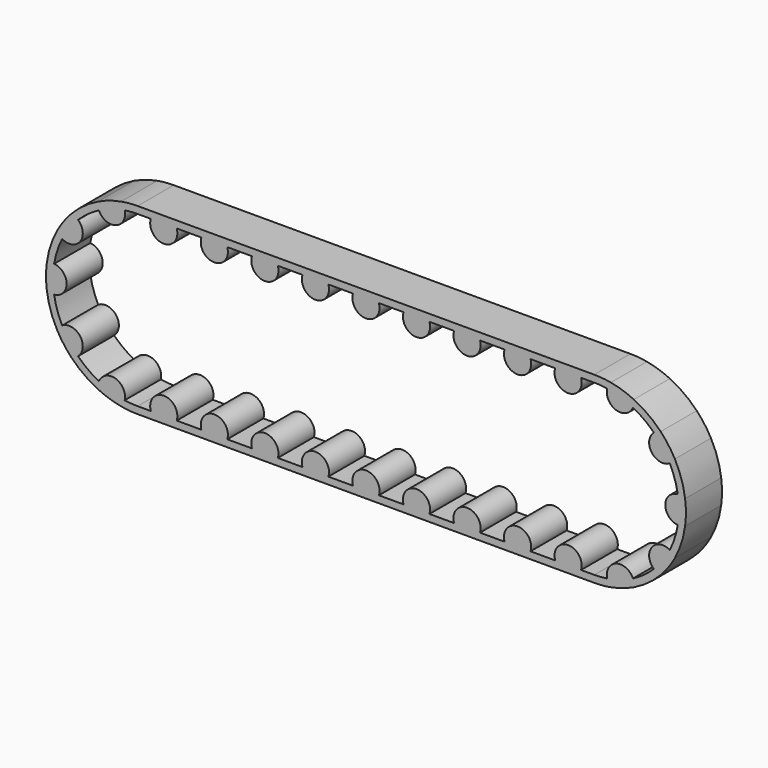
from build123d import *

# Parameters (mm, degrees)
F3_DEPTH     = 25.4
F4_TEXT_SIZE = 22.0144093166
F5_DEPTH     = 2.54


# Not quite as in the source:
# - Text() gives the source's letters only with a copy of the font that has no kerning and outlines rounded to 1/6400 em; it was checked with that copy


with BuildPart() as f3:
    # F2 (on Front) → F3 (new body)
    with BuildSketch(Plane.XZ):
        with BuildLine():
            Line((7.4325236662, -47.625), (0, -47.625))
            ThreePointArc((0, -47.625), (-3.6490858874, -47.4849954953), (-7.2767171413, -47.0658051312))
            ThreePointArc((-7.2767171413, -47.0658051312), (-8.0516506043, -49.0450507496), (-9.3413778335, -50.7345887825))
            ThreePointArc((-9.3413778335, -50.7345887825), (-4.6901126532, -51.3737547981), (0, -51.5874))
            Line((0, -51.5874), (10.3706895119, -51.5874))
            ThreePointArc((10.3706895119, -51.5874), (8.5733856685, -49.8495796433), (7.4325236662, -47.625))
        make_face()
        with BuildLine():
            ThreePointArc((-9.3413778335, -50.7345887825), (-8.0516506043, -49.0450507496), (-7.2767171413, -47.0658051312))
            ThreePointArc((-7.2767171413, -47.0658051312), (-14.7169343571, -45.2940665886), (-21.7775983128, -42.3541832258))
            ThreePointArc((-21.7775983128, -42.3541832258), (-22.3140353569, -44.4109210282), (-22.2637096494, -46.5358686543))
            ThreePointArc((-22.2637096494, -46.5358686543), (-15.9413832956, -49.0625329287), (-9.3413778335, -50.7345887825))
        make_face()
        with BuildLine():
            Line((22.001345048, -47.625), (7.4325236662, -47.625))
            ThreePointArc((7.4325236662, -47.625), (8.5733856685, -49.8495796433), (10.3706895119, -51.5874))
            Line((10.3706895119, -51.5874), (19.0631792023, -51.5874))
            ThreePointArc((19.0631792023, -51.5874), (20.8604830458, -49.8495796433), (22.001345048, -47.625))
        make_face()
        with BuildLine():
            ThreePointArc((-22.2637096494, -46.5358686543), (-22.3140353569, -44.4109210282), (-21.7775983128, -42.3541832258))
            ThreePointArc((-21.7775983128, -42.3541832258), (-27.9932726404, -38.5294343571), (-33.5515739739, -33.7998891843))
            ThreePointArc((-33.5515739739, -33.7998891843), (-35.3418797002, -34.9456380646), (-37.3783764856, -35.5544204011))
            ThreePointArc((-37.3783764856, -35.5544204011), (-30.3223129241, -41.7350832956), (-22.2637096494, -46.5358686543))
        make_face()
        with BuildLine():
            Line((35.8862447978, -47.625), (22.001345048, -47.625))
            ThreePointArc((22.001345048, -47.625), (20.8604830458, -49.8495796433), (19.0631792023, -51.5874))
            Line((19.0631792023, -51.5874), (38.8244106435, -51.5874))
            ThreePointArc((38.8244106435, -51.5874), (37.0271068, -49.8495796433), (35.8862447978, -47.625))
        make_face()
        with BuildLine():
            ThreePointArc((-37.3783764856, -35.5544204011), (-35.3418797002, -34.9456380646), (-33.5515739739, -33.7998891843))
            ThreePointArc((-33.5515739739, -33.7998891843), (-38.5294343571, -27.9932726404), (-42.5136114048, -21.4647028939))
            ThreePointArc((-42.5136114048, -21.4647028939), (-44.156518238, -22.8133289458), (-45.3648167618, -24.5620283961))
            ThreePointArc((-45.3648167618, -24.5620283961), (-41.7350832956, -30.3223129241), (-37.3783764856, -35.5544204011))
        make_face()
        with BuildLine():
            Line((50.4550661796, -47.625), (35.8862447978, -47.625))
            ThreePointArc((35.8862447978, -47.625), (37.0271068, -49.8495796433), (38.8244106435, -51.5874))
            Line((38.8244106435, -51.5874), (47.5169003339, -51.5874))
            ThreePointArc((47.5169003339, -51.5874), (49.3142041773, -49.8495796433), (50.4550661796, -47.625))
        make_face()
        with BuildLine():
            ThreePointArc((-45.3648167618, -24.5620283961), (-44.156518238, -22.8133289458), (-42.5136114048, -21.4647028939))
            ThreePointArc((-42.5136114048, -21.4647028939), (-45.2940665886, -14.7169343571), (-47.0108699246, -7.623564385))
            ThreePointArc((-47.0108699246, -7.623564385), (-49.132711977, -7.4981793975), (-51.1381057646, -6.7936718767))
            ThreePointArc((-51.1381057646, -6.7936718767), (-49.0625329287, -15.9413832956), (-45.3648167618, -24.5620283961))
        make_face()
        with BuildLine():
            Line((64.3399659294, -47.625), (50.4550661796, -47.625))
            ThreePointArc((50.4550661796, -47.625), (49.3142041773, -49.8495796433), (47.5169003339, -51.5874))
            Line((47.5169003339, -51.5874), (67.278131775, -51.5874))
            ThreePointArc((67.278131775, -51.5874), (65.4808279316, -49.8495796433), (64.3399659294, -47.625))
        make_face()
        with BuildLine():
            ThreePointArc((-51.1381057646, -6.7936718767), (-49.132711977, -7.4981793975), (-47.0108699246, -7.623564385))
            ThreePointArc((-47.0108699246, -7.623564385), (-47.625, 0), (-47.0108699246, 7.623564385))
            ThreePointArc((-47.0108699246, 7.623564385), (-49.132711977, 7.4981793975), (-51.1381057646, 6.7936718767))
            ThreePointArc((-51.1381057646, 6.7936718767), (-51.5874, 0), (-51.1381057646, -6.7936718767))
        make_face()
        with BuildLine():
            Line((78.9087873111, -47.625), (64.3399659294, -47.625))
            ThreePointArc((64.3399659294, -47.625), (65.4808279316, -49.8495796433), (67.278131775, -51.5874))
            Line((67.278131775, -51.5874), (75.9706214655, -51.5874))
            ThreePointArc((75.9706214655, -51.5874), (77.7679253089, -49.8495796433), (78.9087873111, -47.625))
        make_face()
        with BuildLine():
            ThreePointArc((-51.1381057646, 6.7936718767), (-49.132711977, 7.4981793975), (-47.0108699246, 7.623564385))
            ThreePointArc((-47.0108699246, 7.623564385), (-45.2940665886, 14.7169343571), (-42.5136114048, 21.4647028939))
            ThreePointArc((-42.5136114048, 21.4647028939), (-44.156518238, 22.8133289458), (-45.3648167618, 24.5620283961))
            ThreePointArc((-45.3648167618, 24.5620283961), (-49.0625329287, 15.9413832956), (-51.1381057646, 6.7936718767))
        make_face()
        with BuildLine():
            Line((92.7936870609, -47.625), (78.9087873111, -47.625))
            ThreePointArc((78.9087873111, -47.625), (77.7679253089, -49.8495796433), (75.9706214655, -51.5874))
            Line((75.9706214655, -51.5874), (95.7318529066, -51.5874))
            ThreePointArc((95.7318529066, -51.5874), (93.9345490632, -49.8495796433), (92.7936870609, -47.625))
        make_face()
        with BuildLine():
            ThreePointArc((-45.3648167618, 24.5620283961), (-44.156518238, 22.8133289458), (-42.5136114048, 21.4647028939))
            ThreePointArc((-42.5136114048, 21.4647028939), (-38.5294343571, 27.9932726404), (-33.5515739739, 33.7998891843))
            ThreePointArc((-33.5515739739, 33.7998891843), (-35.3418797002, 34.9456380646), (-37.3783764856, 35.5544204011))
            ThreePointArc((-37.3783764856, 35.5544204011), (-41.7350832956, 30.3223129241), (-45.3648167618, 24.5620283961))
        make_face()
        with BuildLine():
            Line((107.3625084427, -47.625), (92.7936870609, -47.625))
            ThreePointArc((92.7936870609, -47.625), (93.9345490632, -49.8495796433), (95.7318529066, -51.5874))
            Line((95.7318529066, -51.5874), (104.424342597, -51.5874))
            ThreePointArc((104.424342597, -51.5874), (106.2216464405, -49.8495796433), (107.3625084427, -47.625))
        make_face()
        with BuildLine():
            ThreePointArc((-37.3783764856, 35.5544204011), (-35.3418797002, 34.9456380646), (-33.5515739739, 33.7998891843))
            ThreePointArc((-33.5515739739, 33.7998891843), (-27.9932726404, 38.5294343571), (-21.7775983128, 42.3541832258))
            ThreePointArc((-21.7775983128, 42.3541832258), (-22.3140353569, 44.4109210282), (-22.2637096494, 46.5358686543))
            ThreePointArc((-22.2637096494, 46.5358686543), (-30.3223129241, 41.7350832956), (-37.3783764856, 35.5544204011))
        make_face()
        with BuildLine():
            Line((121.2474081925, -47.625), (107.3625084427, -47.625))
            ThreePointArc((107.3625084427, -47.625), (106.2216464405, -49.8495796433), (104.424342597, -51.5874))
            Line((104.424342597, -51.5874), (124.1855740382, -51.5874))
            ThreePointArc((124.1855740382, -51.5874), (122.3882701947, -49.8495796433), (121.2474081925, -47.625))
        make_face()
        with BuildLine():
            ThreePointArc((-22.2637096494, 46.5358686543), (-22.3140353569, 44.4109210282), (-21.7775983128, 42.3541832258))
            ThreePointArc((-21.7775983128, 42.3541832258), (-14.7169343571, 45.2940665886), (-7.2767171413, 47.0658051312))
            ThreePointArc((-7.2767171413, 47.0658051312), (-8.0516506043, 49.0450507496), (-9.3413778335, 50.7345887825))
            ThreePointArc((-9.3413778335, 50.7345887825), (-15.9413832956, 49.0625329287), (-22.2637096494, 46.5358686543))
        make_face()
        with BuildLine():
            Line((135.8162295743, -47.625), (121.2474081925, -47.625))
            ThreePointArc((121.2474081925, -47.625), (122.3882701947, -49.8495796433), (124.1855740382, -51.5874))
            Line((124.1855740382, -51.5874), (132.8780637286, -51.5874))
            ThreePointArc((132.8780637286, -51.5874), (134.675367572, -49.8495796433), (135.8162295743, -47.625))
        make_face()
        with BuildLine():
            ThreePointArc((-9.3413778335, 50.7345887825), (-8.0516506043, 49.0450507496), (-7.2767171413, 47.0658051312))
            ThreePointArc((-7.2767171413, 47.0658051312), (-3.6490858874, 47.4849954953), (0, 47.625))
            Line((0, 47.625), (7.4325236662, 47.625))
            ThreePointArc((7.4325236662, 47.625), (8.5733856685, 49.8495796433), (10.3706895119, 51.5874))
            Line((10.3706895119, 51.5874), (0, 51.5874))
            ThreePointArc((0, 51.5874), (-4.6901126532, 51.3737547981), (-9.3413778335, 50.7345887825))
        make_face()
        with BuildLine():
            Line((149.7011293241, -47.625), (135.8162295743, -47.625))
            ThreePointArc((135.8162295743, -47.625), (134.675367572, -49.8495796433), (132.8780637286, -51.5874))
            Line((132.8780637286, -51.5874), (152.6392951697, -51.5874))
            ThreePointArc((152.6392951697, -51.5874), (150.8419913263, -49.8495796433), (149.7011293241, -47.625))
        make_face()
        with BuildLine():
            Line((164.2699507058, -47.625), (149.7011293241, -47.625))
            ThreePointArc((149.7011293241, -47.625), (150.8419913263, -49.8495796433), (152.6392951697, -51.5874))
            Line((152.6392951697, -51.5874), (161.3317848602, -51.5874))
            ThreePointArc((161.3317848602, -51.5874), (163.1290887036, -49.8495796433), (164.2699507058, -47.625))
        make_face()
        with BuildLine():
            ThreePointArc((10.3706895119, 51.5874), (8.5733856685, 49.8495796433), (7.4325236662, 47.625))
            Line((7.4325236662, 47.625), (22.001345048, 47.625))
            ThreePointArc((22.001345048, 47.625), (20.8604830458, 49.8495796433), (19.0631792023, 51.5874))
            Line((19.0631792023, 51.5874), (10.3706895119, 51.5874))
        make_face()
        with BuildLine():
            Line((178.1548504556, -47.625), (164.2699507058, -47.625))
            ThreePointArc((164.2699507058, -47.625), (163.1290887036, -49.8495796433), (161.3317848602, -51.5874))
            Line((161.3317848602, -51.5874), (181.0930163013, -51.5874))
            ThreePointArc((181.0930163013, -51.5874), (179.2957124579, -49.8495796433), (178.1548504556, -47.625))
        make_face()
        with BuildLine():
            ThreePointArc((19.0631792023, 51.5874), (20.8604830458, 49.8495796433), (22.001345048, 47.625))
            Line((22.001345048, 47.625), (35.8862447978, 47.625))
            ThreePointArc((35.8862447978, 47.625), (37.0271068, 49.8495796433), (38.8244106435, 51.5874))
            Line((38.8244106435, 51.5874), (19.0631792023, 51.5874))
        make_face()
        with BuildLine():
            Line((192.7236718374, -47.625), (178.1548504556, -47.625))
            ThreePointArc((178.1548504556, -47.625), (179.2957124579, -49.8495796433), (181.0930163013, -51.5874))
            Line((181.0930163013, -51.5874), (189.7855059917, -51.5874))
            ThreePointArc((189.7855059917, -51.5874), (191.5828098352, -49.8495796433), (192.7236718374, -47.625))
        make_face()
        with BuildLine():
            ThreePointArc((38.8244106435, 51.5874), (37.0271068, 49.8495796433), (35.8862447978, 47.625))
            Line((35.8862447978, 47.625), (50.4550661796, 47.625))
            ThreePointArc((50.4550661796, 47.625), (49.3142041773, 49.8495796433), (47.5169003339, 51.5874))
            Line((47.5169003339, 51.5874), (38.8244106435, 51.5874))
        make_face()
        with BuildLine():
            Line((206.6085715872, -47.625), (192.7236718374, -47.625))
            ThreePointArc((192.7236718374, -47.625), (191.5828098352, -49.8495796433), (189.7855059917, -51.5874))
            Line((189.7855059917, -51.5874), (209.5467374329, -51.5874))
            ThreePointArc((209.5467374329, -51.5874), (207.7494335894, -49.8495796433), (206.6085715872, -47.625))
        make_face()
        with BuildLine():
            ThreePointArc((47.5169003339, 51.5874), (49.3142041773, 49.8495796433), (50.4550661796, 47.625))
            Line((50.4550661796, 47.625), (64.3399659294, 47.625))
            ThreePointArc((64.3399659294, 47.625), (65.4808279316, 49.8495796433), (67.278131775, 51.5874))
            Line((67.278131775, 51.5874), (47.5169003339, 51.5874))
        make_face()
        with BuildLine():
            Line((221.177392969, -47.625), (206.6085715872, -47.625))
            ThreePointArc((206.6085715872, -47.625), (207.7494335894, -49.8495796433), (209.5467374329, -51.5874))
            Line((209.5467374329, -51.5874), (218.2392271233, -51.5874))
            ThreePointArc((218.2392271233, -51.5874), (220.0365309668, -49.8495796433), (221.177392969, -47.625))
        make_face()
        with BuildLine():
            ThreePointArc((67.278131775, 51.5874), (65.4808279316, 49.8495796433), (64.3399659294, 47.625))
            Line((64.3399659294, 47.625), (78.9087873111, 47.625))
            ThreePointArc((78.9087873111, 47.625), (77.7679253089, 49.8495796433), (75.9706214655, 51.5874))
            Line((75.9706214655, 51.5874), (67.278131775, 51.5874))
        make_face()
        with BuildLine():
            Line((235.0622927188, -47.625), (221.177392969, -47.625))
            ThreePointArc((221.177392969, -47.625), (220.0365309668, -49.8495796433), (218.2392271233, -51.5874))
            Line((218.2392271233, -51.5874), (238.0004585645, -51.5874))
            ThreePointArc((238.0004585645, -51.5874), (236.203154721, -49.8495796433), (235.0622927188, -47.625))
        make_face()
        with BuildLine():
            ThreePointArc((75.9706214655, 51.5874), (77.7679253089, 49.8495796433), (78.9087873111, 47.625))
            Line((78.9087873111, 47.625), (92.7936870609, 47.625))
            ThreePointArc((92.7936870609, 47.625), (93.9345490632, 49.8495796433), (95.7318529066, 51.5874))
            Line((95.7318529066, 51.5874), (75.9706214655, 51.5874))
        make_face()
        with BuildLine():
            Line((249.6311141006, -47.625), (235.0622927188, -47.625))
            ThreePointArc((235.0622927188, -47.625), (236.203154721, -49.8495796433), (238.0004585645, -51.5874))
            Line((238.0004585645, -51.5874), (246.6929482549, -51.5874))
            ThreePointArc((246.6929482549, -51.5874), (248.4902520983, -49.8495796433), (249.6311141006, -47.625))
        make_face()
        with BuildLine():
            ThreePointArc((95.7318529066, 51.5874), (93.9345490632, 49.8495796433), (92.7936870609, 47.625))
            Line((92.7936870609, 47.625), (107.3625084427, 47.625))
            ThreePointArc((107.3625084427, 47.625), (106.2216464405, 49.8495796433), (104.424342597, 51.5874))
            Line((104.424342597, 51.5874), (95.7318529066, 51.5874))
        make_face()
        with BuildLine():
            Line((257.0636377668, -47.625), (249.6311141006, -47.625))
            ThreePointArc((249.6311141006, -47.625), (248.4902520983, -49.8495796433), (246.6929482549, -51.5874))
            Line((246.6929482549, -51.5874), (257.0636377668, -51.5874))
            ThreePointArc((257.0636377668, -51.5874), (261.75375042, -51.3737547981), (266.4050156002, -50.7345887825))
            ThreePointArc((266.4050156002, -50.7345887825), (265.1152883711, -49.0450507496), (264.3403549081, -47.0658051312))
            ThreePointArc((264.3403549081, -47.0658051312), (260.7127236542, -47.4849954953), (257.0636377668, -47.625))
        make_face()
        with BuildLine():
            ThreePointArc((104.424342597, 51.5874), (106.2216464405, 49.8495796433), (107.3625084427, 47.625))
            Line((107.3625084427, 47.625), (121.2474081925, 47.625))
            ThreePointArc((121.2474081925, 47.625), (122.3882701947, 49.8495796433), (124.1855740382, 51.5874))
            Line((124.1855740382, 51.5874), (104.424342597, 51.5874))
        make_face()
        with BuildLine():
            ThreePointArc((124.1855740382, 51.5874), (122.3882701947, 49.8495796433), (121.2474081925, 47.625))
            Line((121.2474081925, 47.625), (135.8162295743, 47.625))
            ThreePointArc((135.8162295743, 47.625), (134.675367572, 49.8495796433), (132.8780637286, 51.5874))
            Line((132.8780637286, 51.5874), (124.1855740382, 51.5874))
        make_face()
        with BuildLine():
            ThreePointArc((278.8412360796, -42.3541832258), (271.7805721239, -45.2940665886), (264.3403549081, -47.0658051312))
            ThreePointArc((264.3403549081, -47.0658051312), (265.1152883711, -49.0450507496), (266.4050156002, -50.7345887825))
            ThreePointArc((266.4050156002, -50.7345887825), (273.0050210624, -49.0625329287), (279.3273474161, -46.5358686543))
            ThreePointArc((279.3273474161, -46.5358686543), (279.3776731237, -44.4109210282), (278.8412360796, -42.3541832258))
        make_face()
        with BuildLine():
            ThreePointArc((132.8780637286, 51.5874), (134.675367572, 49.8495796433), (135.8162295743, 47.625))
            Line((135.8162295743, 47.625), (149.7011293241, 47.625))
            Line((149.7011293241, 47.625), (164.2699507058, 47.625))
            ThreePointArc((164.2699507058, 47.625), (163.1290887036, 49.8495796433), (161.3317848602, 51.5874))
            Line((161.3317848602, 51.5874), (132.8780637286, 51.5874))
        make_face()
        with BuildLine():
            ThreePointArc((290.6152117407, -33.7998891843), (285.0569104072, -38.5294343571), (278.8412360796, -42.3541832258))
            ThreePointArc((278.8412360796, -42.3541832258), (279.3776731237, -44.4109210282), (279.3273474161, -46.5358686543))
            ThreePointArc((279.3273474161, -46.5358686543), (287.3859506909, -41.7350832956), (294.4420142524, -35.5544204011))
            ThreePointArc((294.4420142524, -35.5544204011), (292.405517467, -34.9456380646), (290.6152117407, -33.7998891843))
        make_face()
        with BuildLine():
            ThreePointArc((299.5772491715, -21.4647028939), (295.5930721239, -27.9932726404), (290.6152117407, -33.7998891843))
            ThreePointArc((290.6152117407, -33.7998891843), (292.405517467, -34.9456380646), (294.4420142524, -35.5544204011))
            ThreePointArc((294.4420142524, -35.5544204011), (298.7987210624, -30.3223129241), (302.4284545285, -24.5620283961))
            ThreePointArc((302.4284545285, -24.5620283961), (301.2201560047, -22.8133289458), (299.5772491715, -21.4647028939))
        make_face()
        with BuildLine():
            ThreePointArc((161.3317848602, 51.5874), (163.1290887036, 49.8495796433), (164.2699507058, 47.625))
            Line((164.2699507058, 47.625), (178.1548504556, 47.625))
            ThreePointArc((178.1548504556, 47.625), (179.2957124579, 49.8495796433), (181.0930163013, 51.5874))
            Line((181.0930163013, 51.5874), (161.3317848602, 51.5874))
        make_face()
        with BuildLine():
            ThreePointArc((304.0745076914, -7.623564385), (302.3577043553, -14.7169343571), (299.5772491715, -21.4647028939))
            ThreePointArc((299.5772491715, -21.4647028939), (301.2201560047, -22.8133289458), (302.4284545285, -24.5620283961))
            ThreePointArc((302.4284545285, -24.5620283961), (306.1261706955, -15.9413832956), (308.2017435314, -6.7936718767))
            ThreePointArc((308.2017435314, -6.7936718767), (306.1963497437, -7.4981793975), (304.0745076914, -7.623564385))
        make_face()
        with BuildLine():
            ThreePointArc((181.0930163013, 51.5874), (179.2957124579, 49.8495796433), (178.1548504556, 47.625))
            Line((178.1548504556, 47.625), (192.7236718374, 47.625))
            ThreePointArc((192.7236718374, 47.625), (191.5828098352, 49.8495796433), (189.7855059917, 51.5874))
            Line((189.7855059917, 51.5874), (181.0930163013, 51.5874))
        make_face()
        with BuildLine():
            ThreePointArc((304.0745076914, 7.623564385), (304.6886377668, 0), (304.0745076914, -7.623564385))
            ThreePointArc((304.0745076914, -7.623564385), (306.1963497437, -7.4981793975), (308.2017435314, -6.7936718767))
            ThreePointArc((308.2017435314, -6.7936718767), (308.6510377668, 0), (308.2017435314, 6.7936718767))
            ThreePointArc((308.2017435314, 6.7936718767), (306.1963497437, 7.4981793975), (304.0745076914, 7.623564385))
        make_face()
        with BuildLine():
            ThreePointArc((189.7855059917, 51.5874), (191.5828098352, 49.8495796433), (192.7236718374, 47.625))
            Line((192.7236718374, 47.625), (206.6085715872, 47.625))
            ThreePointArc((206.6085715872, 47.625), (207.7494335894, 49.8495796433), (209.5467374329, 51.5874))
            Line((209.5467374329, 51.5874), (189.7855059917, 51.5874))
        make_face()
        with BuildLine():
            ThreePointArc((299.5772491715, 21.4647028939), (302.3577043553, 14.7169343571), (304.0745076914, 7.623564385))
            ThreePointArc((304.0745076914, 7.623564385), (306.1963497437, 7.4981793975), (308.2017435314, 6.7936718767))
            ThreePointArc((308.2017435314, 6.7936718767), (306.1261706955, 15.9413832956), (302.4284545285, 24.5620283961))
            ThreePointArc((302.4284545285, 24.5620283961), (301.2201560047, 22.8133289458), (299.5772491715, 21.4647028939))
        make_face()
        with BuildLine():
            ThreePointArc((209.5467374329, 51.5874), (207.7494335894, 49.8495796433), (206.6085715872, 47.625))
            Line((206.6085715872, 47.625), (221.177392969, 47.625))
            ThreePointArc((221.177392969, 47.625), (220.0365309668, 49.8495796433), (218.2392271233, 51.5874))
            Line((218.2392271233, 51.5874), (209.5467374329, 51.5874))
        make_face()
        with BuildLine():
            ThreePointArc((290.6152117407, 33.7998891843), (295.5930721239, 27.9932726404), (299.5772491715, 21.4647028939))
            ThreePointArc((299.5772491715, 21.4647028939), (301.2201560047, 22.8133289458), (302.4284545285, 24.5620283961))
            ThreePointArc((302.4284545285, 24.5620283961), (298.7987210624, 30.3223129241), (294.4420142524, 35.5544204011))
            ThreePointArc((294.4420142524, 35.5544204011), (292.405517467, 34.9456380646), (290.6152117407, 33.7998891843))
        make_face()
        with BuildLine():
            ThreePointArc((218.2392271233, 51.5874), (220.0365309668, 49.8495796433), (221.177392969, 47.625))
            Line((221.177392969, 47.625), (235.0622927188, 47.625))
            ThreePointArc((235.0622927188, 47.625), (236.203154721, 49.8495796433), (238.0004585645, 51.5874))
            Line((238.0004585645, 51.5874), (218.2392271233, 51.5874))
        make_face()
        with BuildLine():
            ThreePointArc((278.8412360796, 42.3541832258), (285.0569104072, 38.5294343571), (290.6152117407, 33.7998891843))
            ThreePointArc((290.6152117407, 33.7998891843), (292.405517467, 34.9456380646), (294.4420142524, 35.5544204011))
            ThreePointArc((294.4420142524, 35.5544204011), (287.3859506909, 41.7350832956), (279.3273474161, 46.5358686543))
            ThreePointArc((279.3273474161, 46.5358686543), (279.3776731237, 44.4109210282), (278.8412360796, 42.3541832258))
        make_face()
        with BuildLine():
            ThreePointArc((238.0004585645, 51.5874), (236.203154721, 49.8495796433), (235.0622927188, 47.625))
            Line((235.0622927188, 47.625), (249.6311141006, 47.625))
            ThreePointArc((249.6311141006, 47.625), (248.4902520983, 49.8495796433), (246.6929482549, 51.5874))
            Line((246.6929482549, 51.5874), (238.0004585645, 51.5874))
        make_face()
        with BuildLine():
            ThreePointArc((264.3403549081, 47.0658051312), (271.7805721239, 45.2940665886), (278.8412360796, 42.3541832258))
            ThreePointArc((278.8412360796, 42.3541832258), (279.3776731237, 44.4109210282), (279.3273474161, 46.5358686543))
            ThreePointArc((279.3273474161, 46.5358686543), (273.0050210624, 49.0625329287), (266.4050156002, 50.7345887825))
            ThreePointArc((266.4050156002, 50.7345887825), (265.1152883711, 49.0450507496), (264.3403549081, 47.0658051312))
        make_face()
        with BuildLine():
            ThreePointArc((246.6929482549, 51.5874), (248.4902520983, 49.8495796433), (249.6311141006, 47.625))
            Line((249.6311141006, 47.625), (257.0636377668, 47.625))
            ThreePointArc((257.0636377668, 47.625), (260.7127236542, 47.4849954953), (264.3403549081, 47.0658051312))
            ThreePointArc((264.3403549081, 47.0658051312), (265.1152883711, 49.0450507496), (266.4050156002, 50.7345887825))
            ThreePointArc((266.4050156002, 50.7345887825), (261.75375042, 51.3737547981), (257.0636377668, 51.5874))
            Line((257.0636377668, 51.5874), (246.6929482549, 51.5874))
        make_face()
        with BuildLine():
            ThreePointArc((-21.7775983128, -42.3541832258), (-14.7169343571, -45.2940665886), (-7.2767171413, -47.0658051312))
            ThreePointArc((-7.2767171413, -47.0658051312), (-12.3534918649, -38.0201385391), (-21.7775983128, -42.3541832258))
        make_face()
        with BuildLine():
            ThreePointArc((22.001345048, -47.625), (14.7169343571, -37.6458060228), (7.4325236662, -47.625))
            Line((7.4325236662, -47.625), (22.001345048, -47.625))
        make_face()
        with BuildLine():
            ThreePointArc((50.4550661796, -47.625), (43.1706554887, -37.6458060228), (35.8862447978, -47.625))
            Line((35.8862447978, -47.625), (50.4550661796, -47.625))
        make_face()
        with BuildLine():
            ThreePointArc((78.9087873111, -47.625), (71.6243766202, -37.6458060228), (64.3399659294, -47.625))
            Line((64.3399659294, -47.625), (78.9087873111, -47.625))
        make_face()
        with BuildLine():
            ThreePointArc((107.3625084427, -47.625), (100.0780977518, -37.6458060228), (92.7936870609, -47.625))
            Line((92.7936870609, -47.625), (107.3625084427, -47.625))
        make_face()
        with BuildLine():
            ThreePointArc((135.8162295743, -47.625), (128.5318188834, -37.6458060228), (121.2474081925, -47.625))
            Line((121.2474081925, -47.625), (135.8162295743, -47.625))
        make_face()
        with BuildLine():
            ThreePointArc((164.2699507058, -47.625), (156.985540015, -37.6458060228), (149.7011293241, -47.625))
            Line((149.7011293241, -47.625), (164.2699507058, -47.625))
        make_face()
        with BuildLine():
            ThreePointArc((192.7236718374, -47.625), (185.4392611465, -37.6458060228), (178.1548504556, -47.625))
            Line((178.1548504556, -47.625), (192.7236718374, -47.625))
        make_face()
        with BuildLine():
            ThreePointArc((221.177392969, -47.625), (213.8929822781, -37.6458060228), (206.6085715872, -47.625))
            Line((206.6085715872, -47.625), (221.177392969, -47.625))
        make_face()
        with BuildLine():
            ThreePointArc((249.6311141006, -47.625), (242.3467034097, -37.6458060228), (235.0622927188, -47.625))
            Line((235.0622927188, -47.625), (249.6311141006, -47.625))
        make_face()
        with BuildLine():
            ThreePointArc((278.8412360796, -42.3541832258), (269.4171296316, -38.0201385391), (264.3403549081, -47.0658051312))
            ThreePointArc((264.3403549081, -47.0658051312), (271.7805721239, -45.2940665886), (278.8412360796, -42.3541832258))
        make_face()
        with BuildLine():
            Line((22.001345048, 47.625), (7.4325236662, 47.625))
            ThreePointArc((7.4325236662, 47.625), (14.7169343571, 37.6458060228), (22.001345048, 47.625))
        make_face()
        with BuildLine():
            ThreePointArc((-7.2767171413, 47.0658051312), (-14.7169343571, 45.2940665886), (-21.7775983128, 42.3541832258))
            ThreePointArc((-21.7775983128, 42.3541832258), (-12.3534918649, 38.0201385391), (-7.2767171413, 47.0658051312))
        make_face()
        with BuildLine():
            ThreePointArc((-33.5515739739, 33.7998891843), (-38.5294343571, 27.9932726404), (-42.5136114048, 21.4647028939))
            ThreePointArc((-42.5136114048, 21.4647028939), (-32.341861582, 23.4977378742), (-33.5515739739, 33.7998891843))
        make_face()
        with BuildLine():
            ThreePointArc((-47.0108699246, 7.623564385), (-47.625, 0), (-47.0108699246, -7.623564385))
            ThreePointArc((-47.0108699246, -7.623564385), (-39.9767394342, 0), (-47.0108699246, 7.623564385))
        make_face()
        with BuildLine():
            ThreePointArc((-42.5136114048, -21.4647028939), (-38.5294343571, -27.9932726404), (-33.5515739739, -33.7998891843))
            ThreePointArc((-33.5515739739, -33.7998891843), (-32.341861582, -23.4977378742), (-42.5136114048, -21.4647028939))
        make_face()
        with BuildLine():
            Line((50.4550661796, 47.625), (35.8862447978, 47.625))
            ThreePointArc((35.8862447978, 47.625), (43.1706554887, 37.6458060228), (50.4550661796, 47.625))
        make_face()
        with BuildLine():
            Line((78.9087873111, 47.625), (64.3399659294, 47.625))
            ThreePointArc((64.3399659294, 47.625), (71.6243766202, 37.6458060228), (78.9087873111, 47.625))
        make_face()
        with BuildLine():
            Line((107.3625084427, 47.625), (92.7936870609, 47.625))
            ThreePointArc((92.7936870609, 47.625), (100.0780977518, 37.6458060228), (107.3625084427, 47.625))
        make_face()
        with BuildLine():
            Line((135.8162295743, 47.625), (121.2474081925, 47.625))
            ThreePointArc((121.2474081925, 47.625), (128.5318188834, 37.6458060228), (135.8162295743, 47.625))
        make_face()
        with BuildLine():
            Line((164.2699507058, 47.625), (149.7011293241, 47.625))
            ThreePointArc((149.7011293241, 47.625), (156.985540015, 37.6458060228), (164.2699507058, 47.625))
        make_face()
        with BuildLine():
            Line((192.7236718374, 47.625), (178.1548504556, 47.625))
            ThreePointArc((178.1548504556, 47.625), (185.4392611465, 37.6458060228), (192.7236718374, 47.625))
        make_face()
        with BuildLine():
            Line((221.177392969, 47.625), (206.6085715872, 47.625))
            ThreePointArc((206.6085715872, 47.625), (213.8929822781, 37.6458060228), (221.177392969, 47.625))
        make_face()
        with BuildLine():
            Line((249.6311141006, 47.625), (235.0622927188, 47.625))
            ThreePointArc((235.0622927188, 47.625), (242.3467034097, 37.6458060228), (249.6311141006, 47.625))
        make_face()
        with BuildLine():
            ThreePointArc((264.3403549081, 47.0658051312), (269.4171296316, 38.0201385391), (278.8412360796, 42.3541832258))
            ThreePointArc((278.8412360796, 42.3541832258), (271.7805721239, 45.2940665886), (264.3403549081, 47.0658051312))
        make_face()
        with BuildLine():
            ThreePointArc((290.6152117407, 33.7998891843), (289.4054993488, 23.4977378742), (299.5772491715, 21.4647028939))
            ThreePointArc((299.5772491715, 21.4647028939), (295.5930721239, 27.9932726404), (290.6152117407, 33.7998891843))
        make_face()
        with BuildLine():
            ThreePointArc((304.0745076914, 7.623564385), (297.040377201, 0), (304.0745076914, -7.623564385))
            ThreePointArc((304.0745076914, -7.623564385), (304.6886377668, 0), (304.0745076914, 7.623564385))
        make_face()
        with BuildLine():
            ThreePointArc((299.5772491715, -21.4647028939), (289.4054993488, -23.4977378742), (290.6152117407, -33.7998891843))
            ThreePointArc((290.6152117407, -33.7998891843), (295.5930721239, -27.9932726404), (299.5772491715, -21.4647028939))
        make_face()
    extrude(amount=F3_DEPTH)

    # F4 (on face) → F5 (cut)
    with BuildSketch(Plane(origin=(0, 0, -51.5874), x_dir=(1, 0, 0), z_dir=(0, 0, -1))):
        with Locations((171.0680909455, 3.7135237362)):
            Text('Stern', F4_TEXT_SIZE, font='Open Sans', text_align=(TextAlign.LEFT, TextAlign.BOTTOM))
    extrude(amount=-F5_DEPTH, mode=Mode.SUBTRACT)


solid = f3.part
